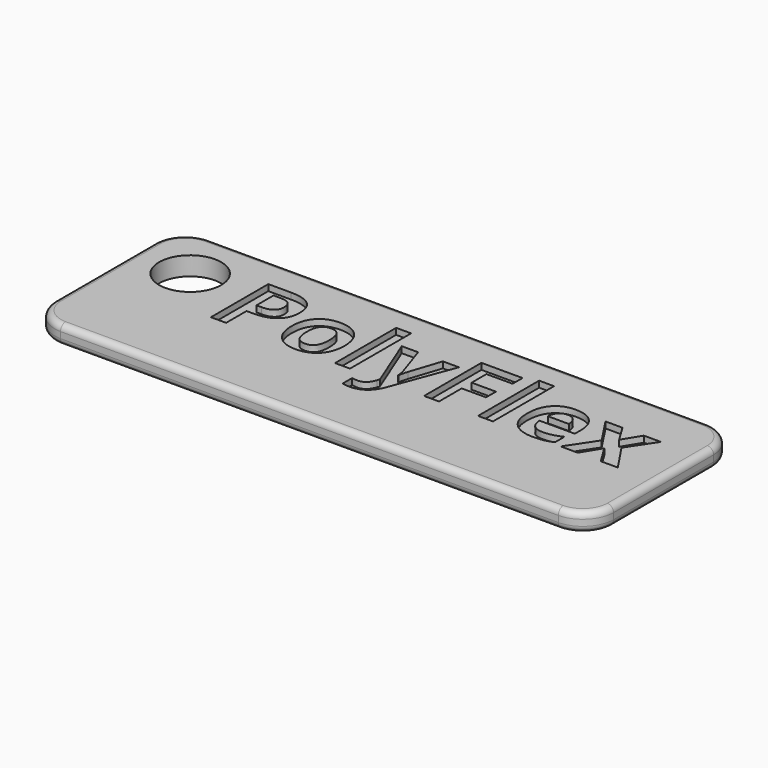
from build123d import *

# Parameters (mm, degrees)
F0_W         = 90
F0_H         = 30
F1_DEPTH     = 3
F2_R         = 1
F3_T3_ANGLE  = 90
F3_T6_ANGLE  = 90
F3_T9_ANGLE  = 90
F3_T12_ANGLE = 90
F3_T15_ANGLE = 90
F3_T18_ANGLE = 90
F3_T21_ANGLE = 90
F3_T24_ANGLE = 90
F3_T27_DEPTH = 3
F3_T30_DEPTH = 3
F3_T33_DEPTH = 3
F3_T36_DEPTH = 3
F4_R         = 5
F5_DEPTH     = 3
F6_TEXT_SIZE = 16.1742297543
F7_DEPTH     = 1


# Not quite as in the source:
# - a fillet or chamfer that OpenCascade refuses, or shapes differently, is made with other operations: its cross-section is extruded or revolved along the edge and cut away or added
# - Text() gives the source's letters only with a copy of the font that has no kerning and outlines rounded to 1/6400 em; it was checked with that copy


with BuildPart() as f1:
    # F0 (on Top) → F1 (new body)
    with BuildSketch(Plane.XY):
        Rectangle(F0_W, F0_H)
    extrude(amount=F1_DEPTH)

    # F2
    f2_edges = [f1.edges().sort_by_distance(p)[0] for p in [
        (0, 15, 3),
        (-45, 0, 3),
        (0, -15, 3),
        (45, 0, 3),
        (0, 15, 0),
        (-45, 0, 0),
        (0, -15, 0),
        (45, 0, 0),
    ]]
    fillet(f2_edges, radius=F2_R)

    # F3: fillet of radius 5 on 4 edges, made by hand


with BuildPart() as f3_tool1:
    # F3_s2 → F3_t3 (revolve)
    with BuildSketch(Plane.YZ.offset(-39.9990343146)):
        with BuildLine():
            ThreePointArc((-14.0004, 0), (-14.7075067812, 0.2928932188), (-15.0004, 1))
            Line((-15.0004, 1), (-15.0004, 0))
            Line((-15.0004, 0), (-14.0004, 0))
        make_face()
    revolve(axis=Axis((-39.9990343146, -9.9990343146, 0), (0, 0, -1)), revolution_arc=F3_T3_ANGLE)


with BuildPart() as f3_tool4:
    # F3_s5 → F3_t6 (revolve)
    with BuildSketch(Plane.XZ.offset(9.9990343146)):
        with BuildLine():
            ThreePointArc((-44.0004, 3), (-44.7075067812, 2.7071067812), (-45.0004, 2))
            Line((-45.0004, 2), (-45.0004, 3))
            Line((-45.0004, 3), (-44.0004, 3))
        make_face()
    revolve(axis=Axis((-39.9990343146, -9.9990343146, 3), (0, 0, 1)), revolution_arc=F3_T6_ANGLE)


with BuildPart() as f3_tool7:
    # F3_s8 → F3_t9 (revolve)
    with BuildSketch(Plane.XZ.offset(-9.9990343146)):
        with BuildLine():
            ThreePointArc((-44.0004, 0), (-44.7075067812, 0.2928932188), (-45.0004, 1))
            Line((-45.0004, 1), (-45.0004, 0))
            Line((-45.0004, 0), (-44.0004, 0))
        make_face()
    revolve(axis=Axis((-39.9990343146, 9.9990343146, 0), (0, 0, -1)), revolution_arc=F3_T9_ANGLE)


with BuildPart() as f3_tool10:
    # F3_s11 → F3_t12 (revolve)
    with BuildSketch(Plane.YZ.offset(-39.9990343146)):
        with BuildLine():
            ThreePointArc((14.0004, 3), (14.7075067812, 2.7071067812), (15.0004, 2))
            Line((15.0004, 2), (15.0004, 3))
            Line((15.0004, 3), (14.0004, 3))
        make_face()
    revolve(axis=Axis((-39.9990343146, 9.9990343146, 3), (0, 0, 1)), revolution_arc=F3_T12_ANGLE)


with BuildPart() as f3_tool13:
    # F3_s14 → F3_t15 (revolve)
    with BuildSketch(Plane.YZ.offset(39.9990343146)):
        with BuildLine():
            ThreePointArc((14.0004, 0), (14.7075067812, 0.2928932188), (15.0004, 1))
            Line((15.0004, 1), (15.0004, 0))
            Line((15.0004, 0), (14.0004, 0))
        make_face()
    revolve(axis=Axis((39.9990343146, 9.9990343146, 0), (0, 0, -1)), revolution_arc=F3_T15_ANGLE)


with BuildPart() as f3_tool16:
    # F3_s17 → F3_t18 (revolve)
    with BuildSketch(Plane.XZ.offset(-9.9990343146)):
        with BuildLine():
            ThreePointArc((44.0004, 3), (44.7075067812, 2.7071067812), (45.0004, 2))
            Line((45.0004, 2), (45.0004, 3))
            Line((45.0004, 3), (44.0004, 3))
        make_face()
    revolve(axis=Axis((39.9990343146, 9.9990343146, 3), (0, 0, 1)), revolution_arc=F3_T18_ANGLE)


with BuildPart() as f3_tool19:
    # F3_s20 → F3_t21 (revolve)
    with BuildSketch(Plane.XZ.offset(9.9990343146)):
        with BuildLine():
            ThreePointArc((44.0004, 0), (44.7075067812, 0.2928932188), (45.0004, 1))
            Line((45.0004, 1), (45.0004, 0))
            Line((45.0004, 0), (44.0004, 0))
        make_face()
    revolve(axis=Axis((39.9990343146, -9.9990343146, 0), (0, 0, -1)), revolution_arc=F3_T21_ANGLE)


with BuildPart() as f3_tool22:
    # F3_s23 → F3_t24 (revolve)
    with BuildSketch(Plane.YZ.offset(39.9990343146)):
        with BuildLine():
            ThreePointArc((-14.0004, 3), (-14.7075067812, 2.7071067812), (-15.0004, 2))
            Line((-15.0004, 2), (-15.0004, 3))
            Line((-15.0004, 3), (-14.0004, 3))
        make_face()
    revolve(axis=Axis((39.9990343146, -9.9990343146, 3), (0, 0, 1)), revolution_arc=F3_T24_ANGLE)


with BuildPart() as f3_tool25:
    # F3_s26 → F3_t27 (new body)
    with BuildSketch(Plane.XY):
        with BuildLine():
            ThreePointArc((45.0004, -9.9990343146), (43.5355339059, -13.5355339059), (39.9990343146, -15.0004))
            Line((39.9990343146, -15.0004), (39.9990343146, -15.5005365685))
            ThreePointArc((39.9990343146, -15.5005365685), (42.4995171573, -15.5001365685), (45, -15.5001365685))
            Line((45, -15.5001365685), (45.5001365685, -15))
            ThreePointArc((45.5001365685, -15), (45.5001365685, -12.4995171573), (45.5005365685, -9.9990343146))
            Line((45.5005365685, -9.9990343146), (45.0004, -9.9990343146))
        make_face()
    extrude(amount=F3_T27_DEPTH)


with BuildPart() as f3_tool28:
    # F3_s29 → F3_t30 (new body)
    with BuildSketch(Plane.XY):
        with BuildLine():
            ThreePointArc((39.9990343146, 15.0004), (43.5355339059, 13.5355339059), (45.0004, 9.9990343146))
            Line((45.0004, 9.9990343146), (45.5005365685, 9.9990343146))
            ThreePointArc((45.5005365685, 9.9990343146), (45.5001365685, 12.4995171573), (45.5001365685, 15))
            Line((45.5001365685, 15), (45, 15.5001365685))
            ThreePointArc((45, 15.5001365685), (42.4995171573, 15.5001365685), (39.9990343146, 15.5005365685))
            Line((39.9990343146, 15.5005365685), (39.9990343146, 15.0004))
        make_face()
    extrude(amount=F3_T30_DEPTH)


with BuildPart() as f3_tool31:
    # F3_s32 → F3_t33 (new body)
    with BuildSketch(Plane.XY):
        with BuildLine():
            ThreePointArc((-39.9990343146, 15.0004), (-43.5355339059, 13.5355339059), (-45.0004, 9.9990343146))
            Line((-45.0004, 9.9990343146), (-45.5005365685, 9.9990343146))
            ThreePointArc((-45.5005365685, 9.9990343146), (-45.5001365685, 12.4995171573), (-45.5001365685, 15))
            Line((-45.5001365685, 15), (-45, 15.5001365685))
            ThreePointArc((-45, 15.5001365685), (-42.4995171573, 15.5001365685), (-39.9990343146, 15.5005365685))
            Line((-39.9990343146, 15.5005365685), (-39.9990343146, 15.0004))
        make_face()
    extrude(amount=F3_T33_DEPTH)


with BuildPart() as f3_tool34:
    # F3_s35 → F3_t36 (new body)
    with BuildSketch(Plane.XY):
        with BuildLine():
            ThreePointArc((-45.0004, -9.9990343146), (-43.5355339059, -13.5355339059), (-39.9990343146, -15.0004))
            Line((-39.9990343146, -15.0004), (-39.9990343146, -15.5005365685))
            ThreePointArc((-39.9990343146, -15.5005365685), (-42.4995171573, -15.5001365685), (-45, -15.5001365685))
            Line((-45, -15.5001365685), (-45.5001365685, -15))
            ThreePointArc((-45.5001365685, -15), (-45.5001365685, -12.4995171573), (-45.5005365685, -9.9990343146))
            Line((-45.5005365685, -9.9990343146), (-45.0004, -9.9990343146))
        make_face()
    extrude(amount=F3_T36_DEPTH)


with BuildPart() as f1_1:
    add(f1.part)

    # F3_t37: cut F3_tool1, F3_tool4, F3_tool7, F3_tool10, F3_tool13, F3_tool16, F3_tool19, F3_tool22, F3_tool25, F3_tool28, F3_tool31, F3_tool34
    add([f3_tool1.part, f3_tool4.part, f3_tool7.part, f3_tool10.part, f3_tool13.part, f3_tool16.part, f3_tool19.part, f3_tool22.part, f3_tool25.part, f3_tool28.part, f3_tool31.part, f3_tool34.part], mode=Mode.SUBTRACT)

    # F4 (on face) → F5 (cut)
    with BuildSketch(Plane.XY.offset(3)):
        with Locations((-36, 6)):
            Circle(F4_R)
    extrude(amount=-F5_DEPTH, mode=Mode.SUBTRACT)

    # F6 (on face) → F7 (cut)
    with BuildSketch(Plane.XY.offset(3)):
        with Locations((-28, -1.6454454231)):
            Text('PolyFlex', F6_TEXT_SIZE, font='Open Sans', font_style=FontStyle.BOLD, text_align=(TextAlign.LEFT, TextAlign.BOTTOM))
    extrude(amount=-F7_DEPTH, mode=Mode.SUBTRACT)


solid = f1_1.part
